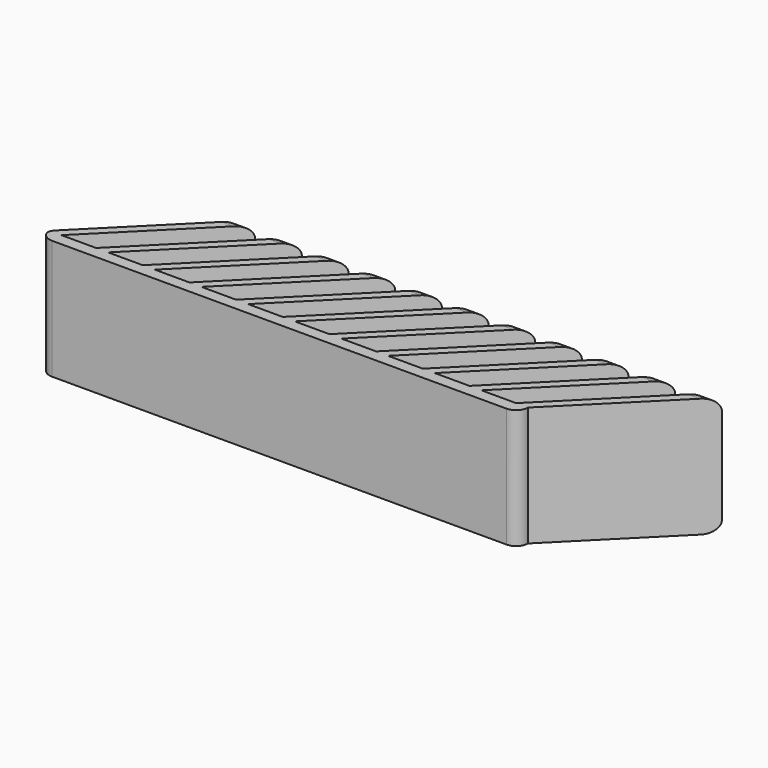
from build123d import *

# Parameters (mm, degrees)
F1_DEPTH     = 25
F2_T1_DEPTH  = 30
F2_T3_DEPTH  = 30
F2_T5_DEPTH  = 30
F2_T7_DEPTH  = 30
F2_T9_DEPTH  = 30
F2_T11_DEPTH = 30
F2_T13_DEPTH = 30
F2_T15_DEPTH = 30
F2_T17_DEPTH = 30
F2_T19_DEPTH = 30
F2_T21_DEPTH = 30
F2_T23_DEPTH = 60.3553390593
F2_T25_DEPTH = 75


# Not quite as in the source:
# - a fillet or chamfer that OpenCascade refuses, or shapes differently, is made with other operations: its cross-section is extruded or revolved along the edge and cut away or added


with BuildPart() as f1:
    # F0 (on Top) → F1 (new body, symmetric)
    with BuildSketch(Plane.XY):
        Polygon((-96.1758106947, -16.0049479455), (-96.1758106947, -21.0049479455), (103.8241893053, -21.0049479455), (103.8241893053, -16.0049479455), (98.8241893053, -16.0049479455), (84.3241893053, -16.0049479455), (79.3241893053, -16.0049479455), (64.8241893053, -16.0049479455), (59.8241893053, -16.0049479455), (45.3241893053, -16.0049479455), (40.3241893053, -16.0049479455), (25.8241893053, -16.0049479455), (20.8241893053, -16.0049479455), (6.3241893053, -16.0049479455), (1.3241893053, -16.0049479455), (-13.1758106947, -16.0049479455), (-18.1758106947, -16.0049479455), (-32.6758106947, -16.0049479455), (-37.6758106947, -16.0049479455), (-52.1758106947, -16.0049479455), (-57.1758106947, -16.0049479455), (-71.6758106947, -16.0049479455), (-76.6758106947, -16.0049479455), (-91.1758106947, -16.0049479455), align=None)
        Polygon((-51.1758106947, 28.9950520545), (-96.1758106947, -16.0049479455), (-91.1758106947, -16.0049479455), (-46.1758106947, 28.9950520545), align=None)
        Polygon((98.8241893053, -16.0049479455), (103.8241893053, -16.0049479455), (148.8241893053, 28.9950520545), (143.8241893053, 28.9950520545), align=None)
        Polygon((-31.6758106947, 28.9950520545), (-76.6758106947, -16.0049479455), (-71.6758106947, -16.0049479455), (-26.6758106947, 28.9950520545), align=None)
        Polygon((79.3241893053, -16.0049479455), (84.3241893053, -16.0049479455), (129.3241893053, 28.9950520545), (124.3241893053, 28.9950520545), align=None)
        Polygon((-12.1758106947, 28.9950520545), (-57.1758106947, -16.0049479455), (-52.1758106947, -16.0049479455), (-7.1758106947, 28.9950520545), align=None)
        Polygon((59.8241893053, -16.0049479455), (64.8241893053, -16.0049479455), (109.8241893053, 28.9950520545), (104.8241893053, 28.9950520545), align=None)
        Polygon((7.3241893053, 28.9950520545), (-37.6758106947, -16.0049479455), (-32.6758106947, -16.0049479455), (12.3241893053, 28.9950520545), align=None)
        Polygon((40.3241893053, -16.0049479455), (45.3241893053, -16.0049479455), (90.3241893053, 28.9950520545), (85.3241893053, 28.9950520545), align=None)
        Polygon((26.8241893053, 28.9950520545), (-18.1758106947, -16.0049479455), (-13.1758106947, -16.0049479455), (31.8241893053, 28.9950520545), align=None)
        Polygon((20.8241893053, -16.0049479455), (25.8241893053, -16.0049479455), (70.8241893053, 28.9950520545), (65.8241893053, 28.9950520545), align=None)
        Polygon((46.3241893053, 28.9950520545), (1.3241893053, -16.0049479455), (6.3241893053, -16.0049479455), (51.3241893053, 28.9950520545), align=None)
    extrude(amount=F1_DEPTH, both=True)

    # F2: fillet of radius 5 on 25 edges, made by hand

    # F2_s2 → F2_t1 (cut)
    with BuildSketch(Plane.YZ.offset(-63.6758106947)):
        with BuildLine():
            ThreePointArc((28.9950520545, 20), (27.5305859605, 23.5355339059), (23.9950520545, 25))
            Line((23.9950520545, 25), (28.9950520545, 25))
            Line((28.9950520545, 25), (28.9950520545, 20))
        make_face()
        with BuildLine():
            ThreePointArc((28.9950520545, -20), (27.5305859605, -23.5355339059), (23.9950520545, -25))
            Line((23.9950520545, -25), (28.9950520545, -25))
            Line((28.9950520545, -25), (28.9950520545, -20))
        make_face()
    extrude(amount=F2_T1_DEPTH, mode=Mode.SUBTRACT)

    # F2_s4 → F2_t3 (cut)
    with BuildSketch(Plane.YZ.offset(-44.1758106947)):
        with BuildLine():
            ThreePointArc((28.9950520545, 20), (27.5305859605, 23.5355339059), (23.9950520545, 25))
            Line((23.9950520545, 25), (28.9950520545, 25))
            Line((28.9950520545, 25), (28.9950520545, 20))
        make_face()
        with BuildLine():
            ThreePointArc((28.9950520545, -20), (27.5305859605, -23.5355339059), (23.9950520545, -25))
            Line((23.9950520545, -25), (28.9950520545, -25))
            Line((28.9950520545, -25), (28.9950520545, -20))
        make_face()
    extrude(amount=F2_T3_DEPTH, mode=Mode.SUBTRACT)

    # F2_s6 → F2_t5 (cut)
    with BuildSketch(Plane.YZ.offset(-24.6758106947)):
        with BuildLine():
            ThreePointArc((28.9950520545, 20), (27.5305859604, 23.5355339059), (23.9950520545, 25))
            Line((23.9950520545, 25), (28.9950520545, 25))
            Line((28.9950520545, 25), (28.9950520545, 20))
        make_face()
        with BuildLine():
            ThreePointArc((28.9950520545, -20), (27.5305859604, -23.5355339059), (23.9950520545, -25))
            Line((23.9950520545, -25), (28.9950520545, -25))
            Line((28.9950520545, -25), (28.9950520545, -20))
        make_face()
    extrude(amount=F2_T5_DEPTH, mode=Mode.SUBTRACT)

    # F2_s8 → F2_t7 (cut)
    with BuildSketch(Plane.YZ.offset(-5.1758106947)):
        with BuildLine():
            ThreePointArc((28.9950520545, 20), (27.5305859604, 23.5355339059), (23.9950520545, 25))
            Line((23.9950520545, 25), (28.9950520545, 25))
            Line((28.9950520545, 25), (28.9950520545, 20))
        make_face()
        with BuildLine():
            ThreePointArc((28.9950520545, -20), (27.5305859604, -23.5355339059), (23.9950520545, -25))
            Line((23.9950520545, -25), (28.9950520545, -25))
            Line((28.9950520545, -25), (28.9950520545, -20))
        make_face()
    extrude(amount=F2_T7_DEPTH, mode=Mode.SUBTRACT)

    # F2_s10 → F2_t9 (cut)
    with BuildSketch(Plane.YZ.offset(14.3241893053)):
        with BuildLine():
            ThreePointArc((28.9950520545, 20), (27.5305859605, 23.5355339059), (23.9950520545, 25))
            Line((23.9950520545, 25), (28.9950520545, 25))
            Line((28.9950520545, 25), (28.9950520545, 20))
        make_face()
        with BuildLine():
            ThreePointArc((28.9950520545, -20), (27.5305859605, -23.5355339059), (23.9950520545, -25))
            Line((23.9950520545, -25), (28.9950520545, -25))
            Line((28.9950520545, -25), (28.9950520545, -20))
        make_face()
    extrude(amount=F2_T9_DEPTH, mode=Mode.SUBTRACT)

    # F2_s12 → F2_t11 (cut)
    with BuildSketch(Plane.YZ.offset(33.8241893053)):
        with BuildLine():
            ThreePointArc((28.9950520545, 20), (27.5305859605, 23.5355339059), (23.9950520545, 25))
            Line((23.9950520545, 25), (28.9950520545, 25))
            Line((28.9950520545, 25), (28.9950520545, 20))
        make_face()
        with BuildLine():
            ThreePointArc((28.9950520545, -20), (27.5305859605, -23.5355339059), (23.9950520545, -25))
            Line((23.9950520545, -25), (28.9950520545, -25))
            Line((28.9950520545, -25), (28.9950520545, -20))
        make_face()
    extrude(amount=F2_T11_DEPTH, mode=Mode.SUBTRACT)

    # F2_s14 → F2_t13 (cut)
    with BuildSketch(Plane.YZ.offset(53.3241893053)):
        with BuildLine():
            ThreePointArc((28.9950520545, 20), (27.5305859605, 23.5355339059), (23.9950520545, 25))
            Line((23.9950520545, 25), (28.9950520545, 25))
            Line((28.9950520545, 25), (28.9950520545, 20))
        make_face()
        with BuildLine():
            ThreePointArc((28.9950520545, -20), (27.5305859605, -23.5355339059), (23.9950520545, -25))
            Line((23.9950520545, -25), (28.9950520545, -25))
            Line((28.9950520545, -25), (28.9950520545, -20))
        make_face()
    extrude(amount=F2_T13_DEPTH, mode=Mode.SUBTRACT)

    # F2_s16 → F2_t15 (cut)
    with BuildSketch(Plane.YZ.offset(72.8241893053)):
        with BuildLine():
            ThreePointArc((28.9950520545, 20), (27.5305859605, 23.5355339059), (23.9950520545, 25))
            Line((23.9950520545, 25), (28.9950520545, 25))
            Line((28.9950520545, 25), (28.9950520545, 20))
        make_face()
        with BuildLine():
            ThreePointArc((28.9950520545, -20), (27.5305859605, -23.5355339059), (23.9950520545, -25))
            Line((23.9950520545, -25), (28.9950520545, -25))
            Line((28.9950520545, -25), (28.9950520545, -20))
        make_face()
    extrude(amount=F2_T15_DEPTH, mode=Mode.SUBTRACT)

    # F2_s18 → F2_t17 (cut)
    with BuildSketch(Plane.YZ.offset(92.3241893053)):
        with BuildLine():
            ThreePointArc((28.9950520545, 20), (27.5305859605, 23.5355339059), (23.9950520545, 25))
            Line((23.9950520545, 25), (28.9950520545, 25))
            Line((28.9950520545, 25), (28.9950520545, 20))
        make_face()
        with BuildLine():
            ThreePointArc((28.9950520545, -20), (27.5305859605, -23.5355339059), (23.9950520545, -25))
            Line((23.9950520545, -25), (28.9950520545, -25))
            Line((28.9950520545, -25), (28.9950520545, -20))
        make_face()
    extrude(amount=F2_T17_DEPTH, mode=Mode.SUBTRACT)

    # F2_s20 → F2_t19 (cut)
    with BuildSketch(Plane.YZ.offset(111.8241893053)):
        with BuildLine():
            ThreePointArc((28.9950520545, 20), (27.5305859605, 23.5355339059), (23.9950520545, 25))
            Line((23.9950520545, 25), (28.9950520545, 25))
            Line((28.9950520545, 25), (28.9950520545, 20))
        make_face()
        with BuildLine():
            ThreePointArc((28.9950520545, -20), (27.5305859605, -23.5355339059), (23.9950520545, -25))
            Line((23.9950520545, -25), (28.9950520545, -25))
            Line((28.9950520545, -25), (28.9950520545, -20))
        make_face()
    extrude(amount=F2_T19_DEPTH, mode=Mode.SUBTRACT)

    # F2_s22 → F2_t21 (cut)
    with BuildSketch(Plane.YZ.offset(131.3241893053)):
        with BuildLine():
            ThreePointArc((28.9950520545, 20), (27.5305859605, 23.5355339059), (23.9950520545, 25))
            Line((23.9950520545, 25), (28.9950520545, 25))
            Line((28.9950520545, 25), (28.9950520545, 20))
        make_face()
        with BuildLine():
            ThreePointArc((28.9950520545, -20), (27.5305859605, -23.5355339059), (23.9950520545, -25))
            Line((23.9950520545, -25), (28.9950520545, -25))
            Line((28.9950520545, -25), (28.9950520545, -20))
        make_face()
    extrude(amount=F2_T21_DEPTH, mode=Mode.SUBTRACT)

    # F2_s24 → F2_t23 (cut)
    with BuildSketch(Plane.XY.offset(-30.1776695297)):
        with BuildLine():
            ThreePointArc((-96.1758106947, -18.0760157573), (-95.7952083573, -16.1625985955), (-94.7113446006, -14.5404818514))
            Line((-94.7113446006, -14.5404818514), (-96.1758106947, -16.0049479455))
            Line((-96.1758106947, -16.0049479455), (-96.1758106947, -18.0760157573))
        make_face()
    extrude(amount=F2_T23_DEPTH, mode=Mode.SUBTRACT)

    # F2_s26 → F2_t25 (cut)
    with BuildSketch(Plane.XY.offset(-37.5)):
        with BuildLine():
            ThreePointArc((-96.1758106947, -16.0049479455), (-94.7113446006, -19.5404818514), (-91.1758106947, -21.0049479455))
            Line((-91.1758106947, -21.0049479455), (-96.1758106947, -21.0049479455))
            Line((-96.1758106947, -21.0049479455), (-96.1758106947, -16.0049479455))
        make_face()
        with BuildLine():
            ThreePointArc((103.8241893053, -16.0049479455), (102.3597232112, -19.5404818514), (98.8241893053, -21.0049479455))
            Line((98.8241893053, -21.0049479455), (103.8241893053, -21.0049479455))
            Line((103.8241893053, -21.0049479455), (103.8241893053, -16.0049479455))
        make_face()
    extrude(amount=F2_T25_DEPTH, mode=Mode.SUBTRACT)


solid = f1.part
